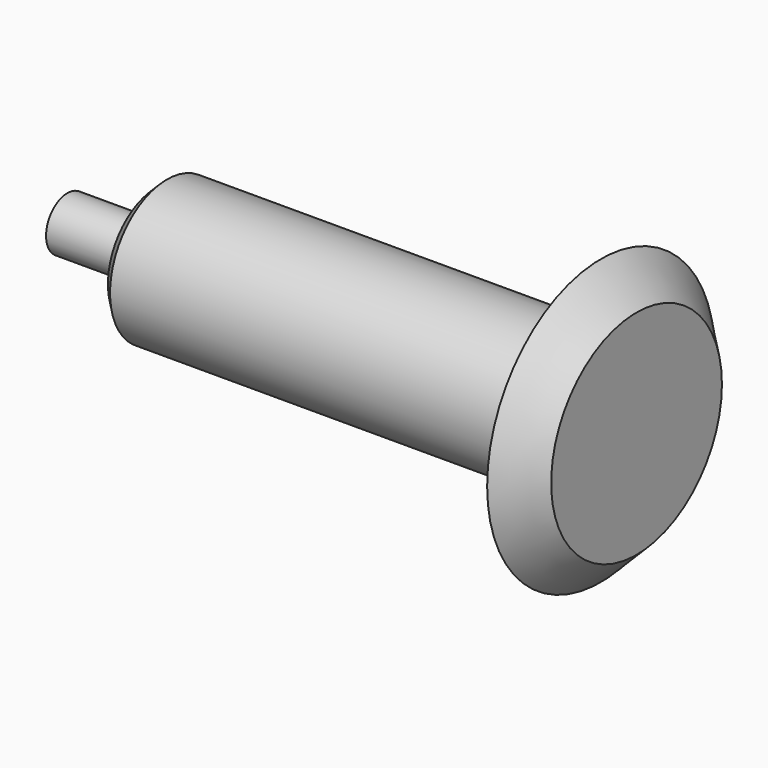
from build123d import *

# Parameters (mm, degrees)
F2_SIZE2 = 10
F2_SIZE  = 10
F3_SIZE2 = 9.99999
F3_SIZE  = 9.99999
F4_SIZE2 = 3
F4_SIZE  = 3


# Not quite as in the source:
# - a fillet or chamfer is up to 0.001 mm smaller than in the source, because OpenCascade refuses the exact size


with BuildPart() as f1:
    # F0 (on Top) → F1 (revolve)
    with BuildSketch(Plane.XY):
        Polygon((-80, 7.5), (-80, 0), (80, 0), (80, 40), (70, 40), (70, 20), (-55, 20), (-55, 7.5), align=None)
    revolve(axis=Axis((0, 0, 0), (-1, 0, 0)))

    # F2
    f2_edges = [f1.edges().sort_by_distance(p)[0] for p in [
        (70, -20, 0),
    ]]
    chamfer(f2_edges, length=F2_SIZE, length2=F2_SIZE2)

    # F3 (size 10 and 10 in the source; OpenCascade refuses exactly that, so slightly less here)
    f3_edges = [f1.edges().sort_by_distance(p)[0] for p in [
        (80, -40, 0),
    ]]
    chamfer(f3_edges, length=F3_SIZE, length2=F3_SIZE2)

    # F4
    f4_edges = [f1.edges().sort_by_distance(p)[0] for p in [
        (-55, -20, 0),
    ]]
    chamfer(f4_edges, length=F4_SIZE, length2=F4_SIZE2)


solid = f1.part
